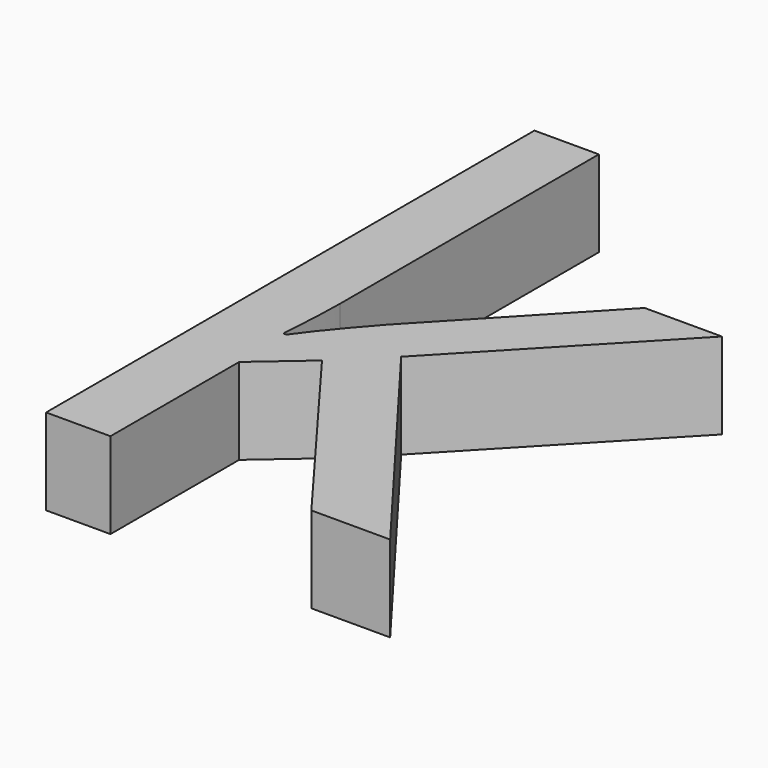
from build123d import *

# Parameters (mm, degrees)
F1_DEPTH = 25.4


with BuildPart() as f1:
    # F0 (on Top) → F1 (new body)
    with BuildSketch(Plane.XY):
        with BuildLine():
            add(Edge.make_bspline(
                [(-480.5364153451, -139.2066991603), (-475.5801438199, -132.1421628818), (-465.4086910628, -120.7131486929)],
                knots=[0, 0, 0, 1, 1, 1], degree=2))
            Line((-480.5364153451, -139.2066991603), (-481.4610928685, -139.2066991603))
            add(Edge.make_bspline(
                [(-480.5364153451, -119.566548564), (-480.5364153451, -125.8913428238), (-481.4610928685, -139.2066991603)],
                knots=[0, 0, 0, 1, 1, 1], degree=2))
            Line((-480.5364153451, -119.566548564), (-480.5364153451, -24.1768152531))
            Line((-480.5364153451, -24.1768152531), (-499.5107981247, -24.1768152531))
            Line((-499.5107981247, -24.1768152531), (-499.5107981247, -204.0450870991))
            Line((-499.5107981247, -204.0450870991), (-480.5364153451, -204.0450870991))
            Line((-480.5364153451, -204.0450870991), (-480.5364153451, -156.6646108016))
            Line((-480.5364153451, -156.6646108016), (-466.1114459806, -144.1629706856))
            Line((-466.1114459806, -144.1629706856), (-421.3570538494, -204.0450870991))
            Line((-421.3570538494, -204.0450870991), (-398.1291544624, -204.0450870991))
            Line((-398.1291544624, -204.0450870991), (-453.0549993506, -131.3284466612))
            Line((-453.0549993506, -131.3284466612), (-401.716903253, -77.3642663973))
            Line((-401.716903253, -77.3642663973), (-424.5009574289, -77.3642663973))
            Line((-424.5009574289, -77.3642663973), (-465.4086910628, -120.7131486929))
        make_face()
    extrude(amount=F1_DEPTH)


solid = f1.part
